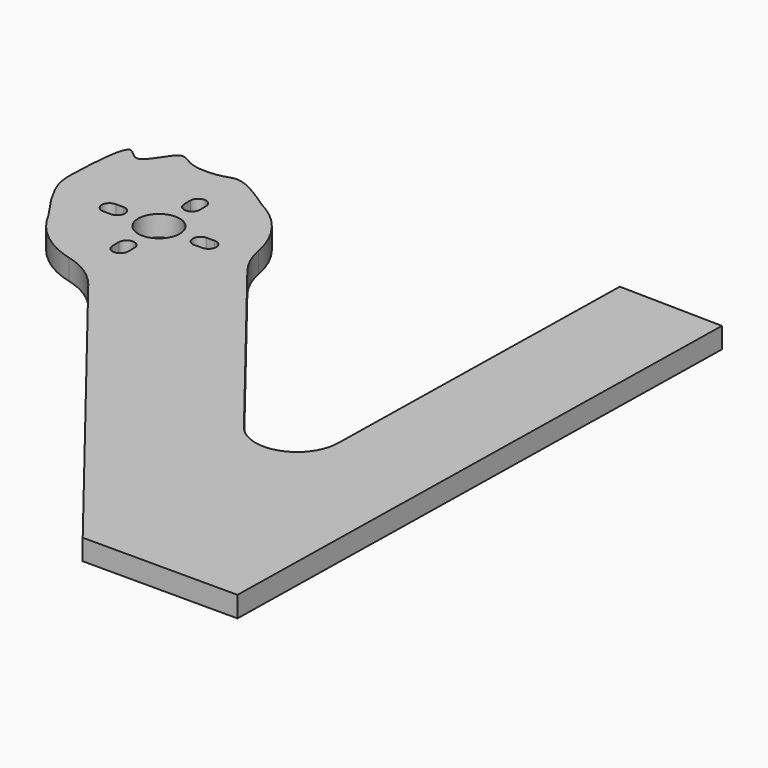
from build123d import *

# Parameters (mm, degrees)
F0_R     = 4
F1_DEPTH = 4


with BuildPart() as f1:
    # F0 (on Top) → F1 (new body)
    with BuildSketch(Plane.XY):
        with BuildLine():
            Line((0, 114.0699429841), (-19.9964126031, 114.4487344947))
            Line((-19.9964126031, 114.4487344947), (-21.2538841411, 48.066782934))
            ThreePointArc((-21.2538841411, 48.066782934), (-26.7144538551, 40.6315624452), (-35.5497771317, 43.284369999))
            Line((-35.5497771317, 43.284369999), (-67.0299300919, 83.4634697431))
            ThreePointArc((-67.0299300919, 83.4634697431), (-68.7751857939, 86.3498052806), (-69.7794614538, 89.5697867556))
            ThreePointArc((-69.7794614538, 89.5697867556), (-71.4485355246, 94.4027474428), (-74.4791847198, 98.5208152801))
            add(Edge.make_bspline(
                [(-78.8449863391, 101.6789579961), (-77.5950408619, 100.8098438948), (-76.1528763386, 99.7673990725), (-74.4791847198, 98.5208152801)],
                knots=[0.9724266933, 0.9724266933, 0.9724266933, 0.9724266933, 1, 1, 1, 1], degree=3))
            ThreePointArc((-78.8449863391, 101.6789579961), (-98.5819159268, 98.459402474), (-101.6001524907, 78.6906853848))
            add(Edge.make_bspline(
                [(-98.5208152802, 74.4791847197), (-99.6937531098, 76.0541274909), (-100.7137627552, 77.4469344608), (-101.6001524907, 78.6906853848)],
                knots=[0, 0, 0, 0, 0.0294140674, 0.0294140674, 0.0294140674, 0.0294140674], degree=3))
            ThreePointArc((-98.5208152802, 74.4791847197), (-94.8707438763, 71.7036948206), (-90.6116540651, 70.0047188308))
            ThreePointArc((-90.6116540651, 70.0047188308), (-86.3811881753, 68.1672164729), (-82.9773982073, 65.0547463263))
            Line((-82.9773982073, 65.0547463263), (-32.007282446, 0))
            Line((-32.007282446, 0), (-2.1608238878, 0))
            Line((-2.1608238878, 0), (0, 114.0699429841))
        make_face()
        with BuildLine():
            Line((-87.9657554412, 77.1471207657), (-87.9712492813, 78.6471585373))
            ThreePointArc((-87.9712492813, 78.6471585373), (-86.4767530063, 80.152642142), (-84.9712694016, 78.658145867))
            Line((-84.9712694016, 78.658145867), (-84.9657755615, 77.1581080954))
            ThreePointArc((-84.9657755615, 77.1581080954), (-86.4602718365, 75.6526244907), (-87.9657554412, 77.1471207657))
        make_face(mode=Mode.SUBTRACT)
        with BuildLine():
            Line((-94.7608149911, 85.0415390363), (-96.2608149911, 85.053518114))
            ThreePointArc((-96.2608149911, 85.053518114), (-97.5661297199, 86.6430647749), (-96.057608469, 88.0412309896))
            Line((-96.057608469, 88.0412309896), (-94.557608469, 88.0292519119))
            ThreePointArc((-94.557608469, 88.0292519119), (-93.0730446096, 86.4275137875), (-94.7608149911, 85.0415390363))
        make_face(mode=Mode.SUBTRACT)
        with Locations((-86.5, 86.4999999999)):
            Circle(F0_R, mode=Mode.SUBTRACT)
        with BuildLine():
            ThreePointArc((-85.0293098025, 94.5054936649), (-86.5238060775, 93.0000100602), (-88.0292896822, 94.4945063352))
            Line((-88.0292896822, 94.4945063352), (-88.0347835222, 95.9945441067))
            ThreePointArc((-88.0347835222, 95.9945441067), (-86.5402872472, 97.5000277114), (-85.0348036425, 96.0055314364))
            Line((-85.0348036425, 96.0055314364), (-85.0293098025, 94.5054936649))
        make_face(mode=Mode.SUBTRACT)
        with BuildLine():
            ThreePointArc((-77.0119786958, 88.0412309896), (-75.5034574448, 86.6430647749), (-76.8087721736, 85.053518114))
            Line((-76.8087721736, 85.053518114), (-78.3087721736, 85.0415390363))
            ThreePointArc((-78.3087721736, 85.0415390363), (-79.9965425552, 86.4275137875), (-78.5119786958, 88.0292519119))
            Line((-78.5119786958, 88.0292519119), (-77.0119786958, 88.0412309896))
        make_face(mode=Mode.SUBTRACT)
        with BuildLine():
            add(Edge.make_bspline(
                [(-78.8449863391, 101.6789579961), (-77.5950408619, 100.8098438948), (-76.1528763386, 99.7673990725), (-74.4791847198, 98.5208152801)],
                knots=[0.9724266933, 0.9724266933, 0.9724266933, 0.9724266933, 1, 1, 1, 1], degree=3))
            ThreePointArc((-74.4791847198, 98.5208152801), (-76.5361640176, 100.2739599431), (-78.8449863391, 101.6789579961))
        make_face()
        with BuildLine():
            ThreePointArc((-101.6001524907, 78.6906853848), (-98.5819159268, 98.459402474), (-78.8449863391, 101.6789579961))
            add(Edge.make_bspline(
                [(-101.6001524907, 78.6906853848), (-107.499308914, 86.9681743468), (-107.4648818789, 89.9713790145), (-106.5144213519, 106.3203180581), (-102.3938787191, 99.2000591205), (-98.758133483, 108.3438184025), (-95.6097715331, 104.6430748676), (-87.2114705595, 104.8772775505), (-86.5984042079, 107.0700769895), (-78.8449863391, 101.6789579961)],
                knots=[0.0294140674, 0.0294140674, 0.0294140674, 0.0294140674, 0.2251724092, 0.3803123381, 0.4666175265, 0.5908143313, 0.6789997688, 0.8013893376, 0.9724266933, 0.9724266933, 0.9724266933, 0.9724266933], degree=3))
        make_face()
        with BuildLine():
            ThreePointArc((-101.6001524907, 78.6906853848), (-100.2230065099, 76.4661028343), (-98.5208152802, 74.4791847197))
            add(Edge.make_bspline(
                [(-98.5208152802, 74.4791847197), (-99.6937531098, 76.0541274909), (-100.7137627552, 77.4469344608), (-101.6001524907, 78.6906853848)],
                knots=[0, 0, 0, 0, 0.0294140674, 0.0294140674, 0.0294140674, 0.0294140674], degree=3))
        make_face()
    extrude(amount=F1_DEPTH)


solid = f1.part
